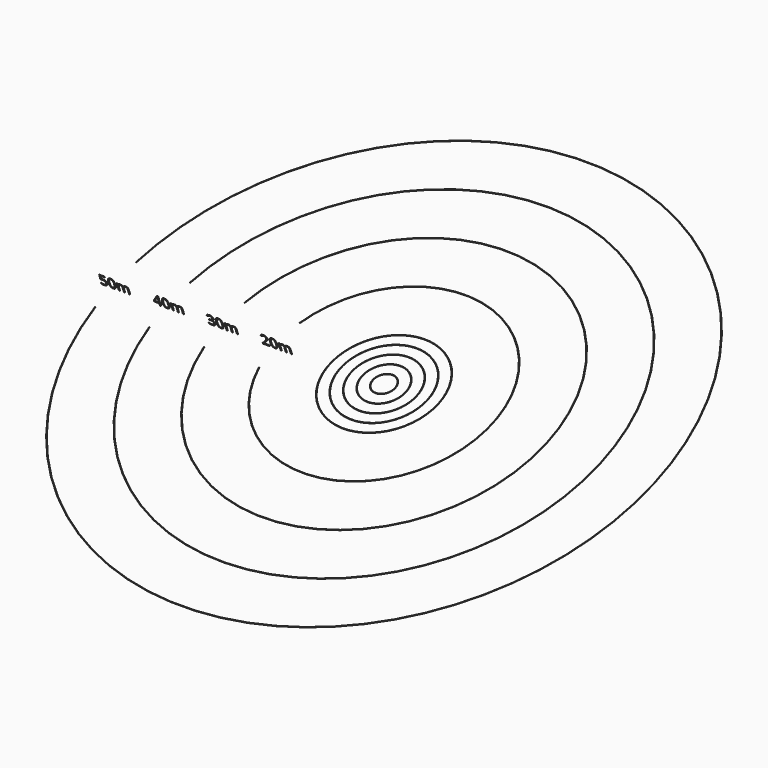
from build123d import *

# Parameters (mm, degrees)
F0_R         = 50100
F0_R_2       = 50000
F0_R_3       = 40100
F0_R_4       = 40000
F0_R_5       = 30100
F0_R_6       = 30000
F0_R_7       = 20100
F0_R_8       = 20000
F0_R_9       = 10100
F0_R_10      = 10000
F0_R_11      = 8100
F0_R_12      = 8000
F0_R_13      = 6100
F0_R_14      = 6000
F0_R_15      = 4100
F0_R_16      = 4000
F0_R_17      = 2100
F0_R_18      = 2000
F1_DEPTH     = 10
F2_W         = 45000
F2_H         = 10000
F3_DEPTH     = 10.001
F4_TEXT_SIZE = 2777.7777777778
F5_DEPTH     = 10
F7_ANGLE     = 90
F8_ANGLE     = 20


# Not quite as in the source:
# - Text() gives the source's letters only with a copy of the font that has no kerning and outlines rounded to 1/6400 em; it was checked with that copy


with BuildPart() as f1:
    # F0 (on Top) → F1 (new body)
    with BuildSketch(Plane.XY):
        Circle(F0_R)
        Circle(F0_R_2, mode=Mode.SUBTRACT)
        Circle(F0_R_3)
        Circle(F0_R_4, mode=Mode.SUBTRACT)
        Circle(F0_R_5)
        Circle(F0_R_6, mode=Mode.SUBTRACT)
        Circle(F0_R_7)
        Circle(F0_R_8, mode=Mode.SUBTRACT)
        Circle(F0_R_9)
        Circle(F0_R_10, mode=Mode.SUBTRACT)
        Circle(F0_R_11)
        Circle(F0_R_12, mode=Mode.SUBTRACT)
        Circle(F0_R_13)
        Circle(F0_R_14, mode=Mode.SUBTRACT)
        Circle(F0_R_15)
        Circle(F0_R_16, mode=Mode.SUBTRACT)
        Circle(F0_R_17)
        Circle(F0_R_18, mode=Mode.SUBTRACT)
    extrude(amount=F1_DEPTH)

    # F2 (on Top) → F3 (cut, through all)
    with BuildSketch(Plane.XY):
        with Locations((-37500, 0)):
            Rectangle(F2_W, F2_H)
    extrude(amount=F3_DEPTH, mode=Mode.SUBTRACT)


with BuildPart() as f5:
    # F4 (on Top) → F5 (new body, through all)
    with BuildSketch(Plane.XY):
        with Locations((-52857.421875, -1000)):
            Text('50m', F4_TEXT_SIZE, font='Open Sans', text_align=(TextAlign.LEFT, TextAlign.BOTTOM))
        with Locations((-42857.421875, -1000)):
            Text('40m', F4_TEXT_SIZE, font='Open Sans', text_align=(TextAlign.LEFT, TextAlign.BOTTOM))
        with Locations((-32857.421875, -1000)):
            Text('30m', F4_TEXT_SIZE, font='Open Sans', text_align=(TextAlign.LEFT, TextAlign.BOTTOM))
        with Locations((-22857.421875, -1000)):
            Text('20m', F4_TEXT_SIZE, font='Open Sans', text_align=(TextAlign.LEFT, TextAlign.BOTTOM))
    extrude(amount=F5_DEPTH)


with BuildPart() as f5_1:
    # F7: moved
    add(f5.part.rotate(Axis((710.9554409981, 0, 0), (1, 0, 0)), F7_ANGLE))


with BuildPart() as f1_1:
    # F8: moved
    add(f1.part.rotate(Axis((710.9554409981, 0, 0), (1, 0, 0)), F8_ANGLE))


with BuildPart() as f5_2:
    # F8: moved
    add(f5_1.part.rotate(Axis((710.9554409981, 0, 0), (1, 0, 0)), F8_ANGLE))


solid = Compound([f1_1.part, f5_2.part])
